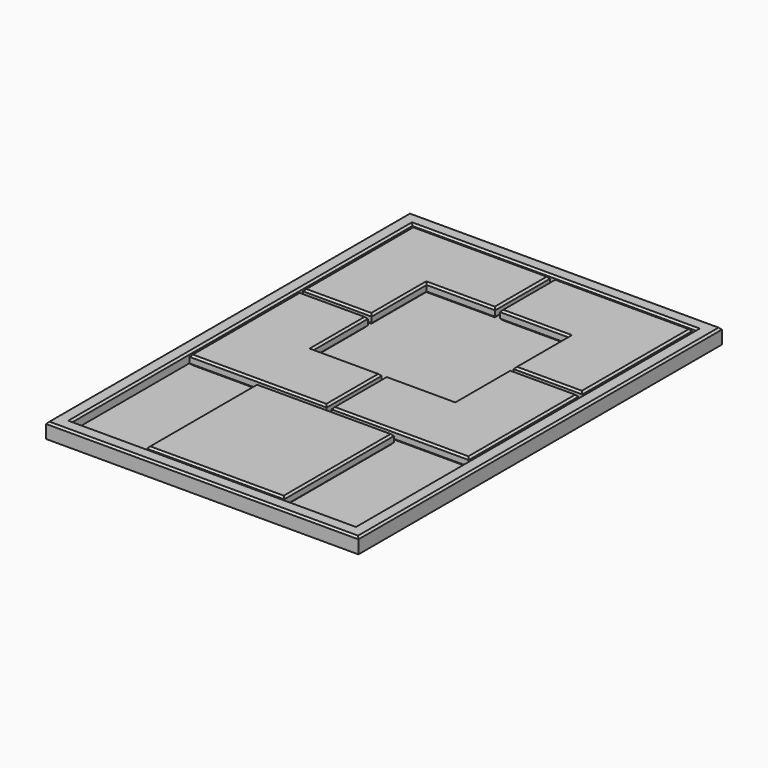
from build123d import *

# Parameters (mm, degrees)
F0_W      = 66
F0_H      = 96
F0_W_2    = 60
F0_H_2    = 90
F1_DEPTH  = 1.2
F2_DEPTH  = 3.2
F4_DEPTH  = 2
F3_W      = 29
F3_H      = 29
F5_SIZE   = 0.4
F5_2_SIZE = 0.4
F5_3_SIZE = 0.4
F5_4_SIZE = 0.4
F5_5_SIZE = 0.4
F5_6_SIZE = 0.4


with BuildPart() as f1:
    # F0 (on Top) → F1 (new body)
    with BuildSketch(Plane.XY):
        Rectangle(F0_W, F0_H)
        Rectangle(F0_W_2, F0_H_2, mode=Mode.SUBTRACT)
        Rectangle(F0_W_2, F0_H_2)
    extrude(amount=F1_DEPTH)

    # F0 (on Top) → F2 (join)
    with BuildSketch(Plane.XY):
        Rectangle(F0_W, F0_H)
        Rectangle(F0_W_2, F0_H_2, mode=Mode.SUBTRACT)
    extrude(amount=F2_DEPTH)

    # F5#6
    f5_6_edges = [f1.edges().sort_by_distance(p)[0] for p in [
        (0, 48, 3.2),
        (-33, 0, 3.2),
        (0, -48, 3.2),
        (33, 0, 3.2),
        (-30, 0, 3.2),
        (0, 45, 3.2),
        (30, 0, 3.2),
        (0, -45, 3.2),
    ]]
    chamfer(f5_6_edges, length=F5_6_SIZE)


with BuildPart() as f4:
    # F3 (on face) → F4 (new body)
    with BuildSketch(Plane.XY.offset(1.2)):
        Polygon((-0.5, 44.5), (-29.5, 44.5), (-29.5, 15.5), (-15, 15.5), (-15, 30), (-0.5, 30), align=None)
    extrude(amount=F4_DEPTH)

    # F5
    f5_edges = [f4.edges().sort_by_distance(p)[0] for p in [
        (-15, 44.5, 3.2),
        (-29.5, 30, 3.2),
        (-22.25, 15.5, 3.2),
        (-15, 22.75, 3.2),
        (-7.75, 30, 3.2),
        (-0.5, 37.25, 3.2),
        (-15, 44.5, 1.2),
        (-29.5, 30, 1.2),
        (-22.25, 15.5, 1.2),
        (-15, 22.75, 1.2),
        (-7.75, 30, 1.2),
        (-0.5, 37.25, 1.2),
    ]]
    chamfer(f5_edges, length=F5_SIZE)


with BuildPart() as f4b:
    # F3 (on face) → F4, piece 2 (new body)
    with BuildSketch(Plane.XY.offset(1.2)):
        Polygon((29.5, 15.5), (29.5, 44.5), (0.5, 44.5), (0.5, 30), (15, 30), (15, 15.5), align=None)
    extrude(amount=F4_DEPTH)

    # F5#2
    f5_2_edges = [f4b.edges().sort_by_distance(p)[0] for p in [
        (29.5, 30, 3.2),
        (15, 44.5, 3.2),
        (0.5, 37.25, 3.2),
        (7.75, 30, 3.2),
        (15, 22.75, 3.2),
        (22.25, 15.5, 3.2),
        (29.5, 30, 1.2),
        (15, 44.5, 1.2),
        (0.5, 37.25, 1.2),
        (7.75, 30, 1.2),
        (15, 22.75, 1.2),
        (22.25, 15.5, 1.2),
    ]]
    chamfer(f5_2_edges, length=F5_2_SIZE)


with BuildPart() as f4c:
    # F3 (on face) → F4, piece 3 (new body)
    with BuildSketch(Plane.XY.offset(1.2)):
        Polygon((-29.5, 14.5), (-29.5, -14.5), (-0.5, -14.5), (-0.5, 0), (-15, 0), (-15, 14.5), align=None)
    extrude(amount=F4_DEPTH)

    # F5#4
    f5_4_edges = [f4c.edges().sort_by_distance(p)[0] for p in [
        (-29.5, 0, 3.2),
        (-15, -14.5, 3.2),
        (-0.5, -7.25, 3.2),
        (-7.75, 0, 3.2),
        (-15, 7.25, 3.2),
        (-22.25, 14.5, 3.2),
        (-29.5, 0, 1.2),
        (-15, -14.5, 1.2),
        (-0.5, -7.25, 1.2),
        (-7.75, 0, 1.2),
        (-15, 7.25, 1.2),
        (-22.25, 14.5, 1.2),
    ]]
    chamfer(f5_4_edges, length=F5_4_SIZE)


with BuildPart() as f4d:
    # F3 (on face) → F4, piece 4 (new body)
    with BuildSketch(Plane.XY.offset(1.2)):
        Polygon((0.5, -14.5), (29.5, -14.5), (29.5, 14.5), (15, 14.5), (15, 0), (0.5, 0), align=None)
    extrude(amount=F4_DEPTH)

    # F5#3
    f5_3_edges = [f4d.edges().sort_by_distance(p)[0] for p in [
        (15, -14.5, 3.2),
        (29.5, 0, 3.2),
        (22.25, 14.5, 3.2),
        (15, 7.25, 3.2),
        (7.75, 0, 3.2),
        (0.5, -7.25, 3.2),
        (15, -14.5, 1.2),
        (29.5, 0, 1.2),
        (22.25, 14.5, 1.2),
        (15, 7.25, 1.2),
        (7.75, 0, 1.2),
        (0.5, -7.25, 1.2),
    ]]
    chamfer(f5_3_edges, length=F5_3_SIZE)


with BuildPart() as f4e:
    # F3 (on face) → F4, piece 5 (new body)
    with BuildSketch(Plane.XY.offset(1.2)):
        with Locations((0, -30)):
            Rectangle(F3_W, F3_H)
    extrude(amount=F4_DEPTH)

    # F5#5
    f5_5_edges = [f4e.edges().sort_by_distance(p)[0] for p in [
        (-14.5, -30, 3.2),
        (0, -44.5, 3.2),
        (14.5, -30, 3.2),
        (0, -15.5, 3.2),
        (-14.5, -30, 1.2),
        (0, -44.5, 1.2),
        (14.5, -30, 1.2),
        (0, -15.5, 1.2),
    ]]
    chamfer(f5_5_edges, length=F5_5_SIZE)


solid = Compound([f1.part, f4.part, f4b.part, f4c.part, f4d.part, f4e.part])
